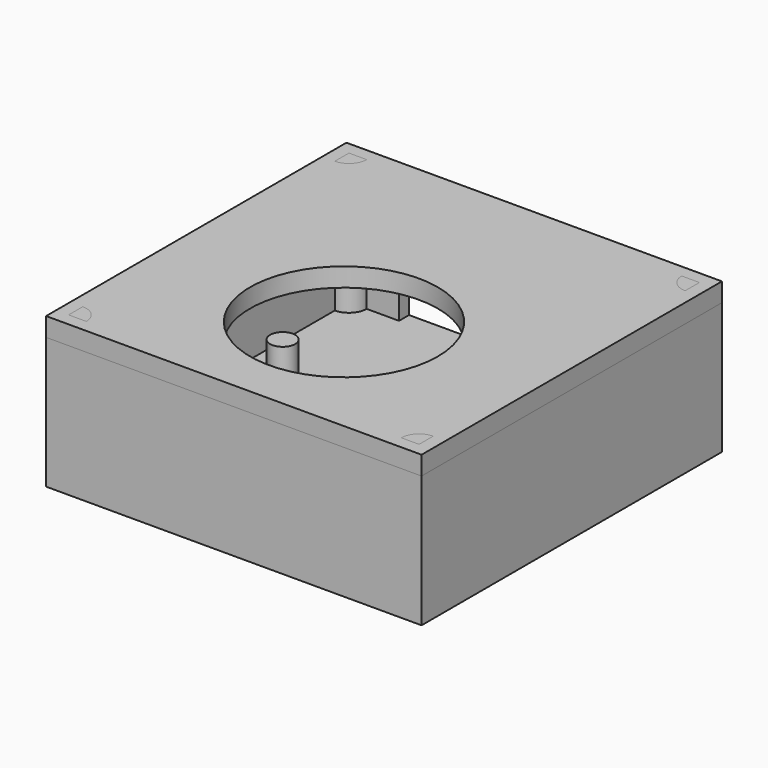
from build123d import *

# Parameters (mm, degrees)
F0_R     = 1
F0_W     = 20
F0_H     = 1
F1_DEPTH = 1.5
F2_DEPTH = 3
F3_DEPTH = 9
F4_W     = 20
F4_H     = 1
F4_R     = 7.5
F5_DEPTH = 1.5
F6_DEPTH = 10.5
F7_DEPTH = 25
F8_DEPTH = 5
F13_R    = 2


with BuildPart() as f1:
    # F0 (on Top) → F1 (new body)
    with BuildSketch(Plane.XY):
        with BuildLine():
            Line((25, -1), (5, -1))
            Line((5, -1), (2.4142135624, -1))
            ThreePointArc((2.4142135624, -1), (2, -2), (1, -2.4142135624))
            Line((1, -2.4142135624), (1, -27.5857864376))
            ThreePointArc((1, -27.5857864376), (2, -28), (2.4142135624, -29))
            Line((2.4142135624, -29), (27.5857864376, -29))
            ThreePointArc((27.5857864376, -29), (28, -28), (29, -27.5857864376))
            Line((29, -27.5857864376), (29, -2.4142135624))
            ThreePointArc((29, -2.4142135624), (28, -2), (27.5857864376, -1))
            Line((27.5857864376, -1), (25, -1))
        make_face()
        with Locations((4.5, -26)):
            Circle(F0_R, mode=Mode.SUBTRACT)
        with Locations((25.5, -26)):
            Circle(F0_R, mode=Mode.SUBTRACT)
        with Locations((4.5, -12)):
            Circle(F0_R, mode=Mode.SUBTRACT)
        with Locations((25.5, -12)):
            Circle(F0_R, mode=Mode.SUBTRACT)
        with BuildLine():
            Line((27.5857864376, -29), (2.4142135624, -29))
            ThreePointArc((2.4142135624, -29), (2.3065629649, -29.5411961001), (2, -30))
            Line((2, -30), (28, -30))
            ThreePointArc((28, -30), (27.6934370351, -29.5411961001), (27.5857864376, -29))
        make_face()
        with BuildLine():
            ThreePointArc((1, -2.4142135624), (0.4588038999, -2.3065629649), (0, -2))
            Line((0, -2), (0, -28))
            ThreePointArc((0, -28), (0.4588038999, -27.6934370351), (1, -27.5857864376))
            Line((1, -27.5857864376), (1, -2.4142135624))
        make_face()
        with BuildLine():
            Line((30, -28), (30, -2))
            ThreePointArc((30, -2), (29.5411961001, -2.3065629649), (29, -2.4142135624))
            Line((29, -2.4142135624), (29, -27.5857864376))
            ThreePointArc((29, -27.5857864376), (29.5411961001, -27.6934370351), (30, -28))
        make_face()
        with Locations((15, -0.5)):
            Rectangle(F0_W, F0_H)
        with BuildLine():
            ThreePointArc((1, -27.5857864376), (0.4588038999, -27.6934370351), (0, -28))
            Line((0, -28), (0, -30))
            Line((0, -30), (2, -30))
            ThreePointArc((2, -30), (2.3065629649, -29.5411961001), (2.4142135624, -29))
            Line((2.4142135624, -29), (1, -29))
            Line((1, -29), (1, -27.5857864376))
        make_face()
        with BuildLine():
            Line((30, -30), (30, -28))
            ThreePointArc((30, -28), (29.5411961001, -27.6934370351), (29, -27.5857864376))
            Line((29, -27.5857864376), (29, -29))
            Line((29, -29), (27.5857864376, -29))
            ThreePointArc((27.5857864376, -29), (27.6934370351, -29.5411961001), (28, -30))
            Line((28, -30), (30, -30))
        make_face()
        with BuildLine():
            ThreePointArc((2.4142135624, -1), (2.3065629649, -0.4588038999), (2, 0))
            Line((2, 0), (0, 0))
            Line((0, 0), (0, -2))
            ThreePointArc((0, -2), (0.4588038999, -2.3065629649), (1, -2.4142135624))
            Line((1, -2.4142135624), (1, -1))
            Line((1, -1), (2.4142135624, -1))
        make_face()
        with BuildLine():
            Line((30, 0), (28, 0))
            ThreePointArc((28, 0), (27.6934370351, -0.4588038999), (27.5857864376, -1))
            Line((27.5857864376, -1), (29, -1))
            Line((29, -1), (29, -2.4142135624))
            ThreePointArc((29, -2.4142135624), (29.5411961001, -2.3065629649), (30, -2))
            Line((30, -2), (30, 0))
        make_face()
        with Locations((4.5, -12)):
            Circle(F0_R)
        with Locations((4.5, -26)):
            Circle(F0_R)
        with Locations((25.5, -26)):
            Circle(F0_R)
        with Locations((25.5, -12)):
            Circle(F0_R)
        with BuildLine():
            Line((28, 0), (25, 0))
            Line((25, 0), (25, -1))
            Line((25, -1), (27.5857864376, -1))
            ThreePointArc((27.5857864376, -1), (27.6934370351, -0.4588038999), (28, 0))
        make_face()
        with BuildLine():
            Line((5, -1), (5, 0))
            Line((5, 0), (2, 0))
            ThreePointArc((2, 0), (2.3065629649, -0.4588038999), (2.4142135624, -1))
            Line((2.4142135624, -1), (5, -1))
        make_face()
        with BuildLine():
            ThreePointArc((1, -2.4142135624), (2, -2), (2.4142135624, -1))
            Line((2.4142135624, -1), (1, -1))
            Line((1, -1), (1, -2.4142135624))
        make_face()
        with BuildLine():
            ThreePointArc((2.4142135624, -29), (2, -28), (1, -27.5857864376))
            Line((1, -27.5857864376), (1, -29))
            Line((1, -29), (2.4142135624, -29))
        make_face()
        with BuildLine():
            Line((29, -29), (29, -27.5857864376))
            ThreePointArc((29, -27.5857864376), (28, -28), (27.5857864376, -29))
            Line((27.5857864376, -29), (29, -29))
        make_face()
        with BuildLine():
            Line((29, -1), (27.5857864376, -1))
            ThreePointArc((27.5857864376, -1), (28, -2), (29, -2.4142135624))
            Line((29, -2.4142135624), (29, -1))
        make_face()
    extrude(amount=-F1_DEPTH)

    # F0 (on Top) → F2 (join)
    with BuildSketch(Plane.XY):
        with Locations((4.5, -12)):
            Circle(F0_R)
        with Locations((25.5, -12)):
            Circle(F0_R)
        with Locations((25.5, -26)):
            Circle(F0_R)
        with Locations((4.5, -26)):
            Circle(F0_R)
    extrude(amount=F2_DEPTH)

    # F0 (on Top) → F3 (join)
    with BuildSketch(Plane.XY):
        with BuildLine():
            ThreePointArc((1, -27.5857864376), (0.4588038999, -27.6934370351), (0, -28))
            Line((0, -28), (0, -30))
            Line((0, -30), (2, -30))
            ThreePointArc((2, -30), (2.3065629649, -29.5411961001), (2.4142135624, -29))
            Line((2.4142135624, -29), (1, -29))
            Line((1, -29), (1, -27.5857864376))
        make_face()
        with BuildLine():
            Line((27.5857864376, -29), (2.4142135624, -29))
            ThreePointArc((2.4142135624, -29), (2.3065629649, -29.5411961001), (2, -30))
            Line((2, -30), (28, -30))
            ThreePointArc((28, -30), (27.6934370351, -29.5411961001), (27.5857864376, -29))
        make_face()
        with BuildLine():
            Line((30, -30), (30, -28))
            ThreePointArc((30, -28), (29.5411961001, -27.6934370351), (29, -27.5857864376))
            Line((29, -27.5857864376), (29, -29))
            Line((29, -29), (27.5857864376, -29))
            ThreePointArc((27.5857864376, -29), (27.6934370351, -29.5411961001), (28, -30))
            Line((28, -30), (30, -30))
        make_face()
        with BuildLine():
            Line((30, -28), (30, -2))
            ThreePointArc((30, -2), (29.5411961001, -2.3065629649), (29, -2.4142135624))
            Line((29, -2.4142135624), (29, -27.5857864376))
            ThreePointArc((29, -27.5857864376), (29.5411961001, -27.6934370351), (30, -28))
        make_face()
        with BuildLine():
            Line((30, 0), (28, 0))
            ThreePointArc((28, 0), (27.6934370351, -0.4588038999), (27.5857864376, -1))
            Line((27.5857864376, -1), (29, -1))
            Line((29, -1), (29, -2.4142135624))
            ThreePointArc((29, -2.4142135624), (29.5411961001, -2.3065629649), (30, -2))
            Line((30, -2), (30, 0))
        make_face()
        with BuildLine():
            Line((28, 0), (25, 0))
            Line((25, 0), (25, -1))
            Line((25, -1), (27.5857864376, -1))
            ThreePointArc((27.5857864376, -1), (27.6934370351, -0.4588038999), (28, 0))
        make_face()
        with BuildLine():
            Line((5, -1), (5, 0))
            Line((5, 0), (2, 0))
            ThreePointArc((2, 0), (2.3065629649, -0.4588038999), (2.4142135624, -1))
            Line((2.4142135624, -1), (5, -1))
        make_face()
        with BuildLine():
            ThreePointArc((2.4142135624, -1), (2.3065629649, -0.4588038999), (2, 0))
            Line((2, 0), (0, 0))
            Line((0, 0), (0, -2))
            ThreePointArc((0, -2), (0.4588038999, -2.3065629649), (1, -2.4142135624))
            Line((1, -2.4142135624), (1, -1))
            Line((1, -1), (2.4142135624, -1))
        make_face()
        with BuildLine():
            ThreePointArc((1, -2.4142135624), (0.4588038999, -2.3065629649), (0, -2))
            Line((0, -2), (0, -28))
            ThreePointArc((0, -28), (0.4588038999, -27.6934370351), (1, -27.5857864376))
            Line((1, -27.5857864376), (1, -2.4142135624))
        make_face()
    extrude(amount=F3_DEPTH)

    # F0 (on Top) → F6 (join)
    with BuildSketch(Plane.XY):
        with BuildLine():
            ThreePointArc((1, -2.4142135624), (2, -2), (2.4142135624, -1))
            Line((2.4142135624, -1), (1, -1))
            Line((1, -1), (1, -2.4142135624))
        make_face()
        with BuildLine():
            ThreePointArc((2.4142135624, -29), (2, -28), (1, -27.5857864376))
            Line((1, -27.5857864376), (1, -29))
            Line((1, -29), (2.4142135624, -29))
        make_face()
        with BuildLine():
            Line((29, -29), (29, -27.5857864376))
            ThreePointArc((29, -27.5857864376), (28, -28), (27.5857864376, -29))
            Line((27.5857864376, -29), (29, -29))
        make_face()
        with BuildLine():
            Line((29, -1), (27.5857864376, -1))
            ThreePointArc((27.5857864376, -1), (28, -2), (29, -2.4142135624))
            Line((29, -2.4142135624), (29, -1))
        make_face()
    extrude(amount=F6_DEPTH)

    # F7 (cut): faces of the model
    f7_faces = [f1.faces().sort_by_distance(p)[0] for p in [
        (28.3997891226, -1.6002108774, 10.5),
        (1.6002108774, -1.6002108774, 10.5),
        (1.6002108774, -28.3997891226, 10.5),
        (28.3997891226, -28.3997891226, 10.5),
    ]]
    extrude(f7_faces, amount=F7_DEPTH, mode=Mode.SUBTRACT)


with BuildPart() as f5:
    # F4 (on face) → F5 (new body)
    with BuildSketch(Plane.XY.offset(9)):
        with Locations((15, -0.5)):
            Rectangle(F4_W, F4_H)
        Polygon((30, 0), (25, 0), (25, -1), (27.5857864376, -1), (29, -1), (29, -2.4142135624), (29, -27.5857864376), (29, -29), (27.5857864376, -29), (2.4142135624, -29), (1, -29), (1, -27.5857864376), (1, -2.4142135624), (1, -1), (2.4142135624, -1), (5, -1), (5, 0), (0, 0), (0, -30), (30, -30), align=None)
        with BuildLine():
            Line((27.5857864376, -1), (25, -1))
            Line((25, -1), (5, -1))
            Line((5, -1), (2.4142135624, -1))
            ThreePointArc((2.4142135624, -1), (2, -2), (1, -2.4142135624))
            Line((1, -2.4142135624), (1, -27.5857864376))
            ThreePointArc((1, -27.5857864376), (2, -28), (2.4142135624, -29))
            Line((2.4142135624, -29), (27.5857864376, -29))
            ThreePointArc((27.5857864376, -29), (28, -28), (29, -27.5857864376))
            Line((29, -27.5857864376), (29, -2.4142135624))
            ThreePointArc((29, -2.4142135624), (28, -2), (27.5857864376, -1))
        make_face()
        with Locations((15, -19)):
            Circle(F4_R, mode=Mode.SUBTRACT)
    extrude(amount=F5_DEPTH)


with BuildPart() as f8:
    # F4 (on face) → F8 (new body)
    with BuildSketch(Plane.XY.offset(9)):
        with Locations((15, -0.5)):
            Rectangle(F4_W, F4_H)
    extrude(amount=-F8_DEPTH)


with BuildPart() as f11:
    # F9 (on Right) → F11 (revolve)
    with BuildSketch(Plane.YZ):
        with BuildLine():
            Line((15.2258750796, -40.7793708146), (25.2258750796, -40.7793708146))
            ThreePointArc((25.2258750796, -40.7793708146), (21.3738474037, -35.9129389037), (15.7530112624, -38.5447591543))
            Line((15.7530112624, -38.5447591543), (9.7055286169, -38.5447591543))
            Line((9.7055286169, -38.5447591543), (9.7055286169, -36.1464507878))
            Line((9.7055286169, -36.1464507878), (5.4970784113, -36.1464507878))
            Line((5.4970784113, -36.1464507878), (5.4970784113, -40.7793708146))
            Line((5.4970784113, -40.7793708146), (15.2258750796, -40.7793708146))
        make_face()
    revolve(axis=Axis((0, 20.2258750796, -40.7793708146), (0, 1, 0)))


with BuildPart() as f12:
    # F10 (on Right) → F12 (revolve)
    with BuildSketch(Plane.YZ):
        with BuildLine():
            ThreePointArc((18.9868118614, -35.8321774343), (23.3636113326, -36.7588470668), (25.3258750796, -40.7793708146))
            Line((25.3258750796, -40.7793708146), (26.2448396534, -40.7793708146))
            Line((26.2448396534, -40.7793708146), (30.2728638053, -40.7793708146))
            Line((30.2728638053, -40.7793708146), (30.2728638053, -38.8744622469))
            Line((30.2728638053, -38.8744622469), (26.2448396534, -38.8744622469))
            Line((26.2448396534, -38.8744622469), (26.2448396534, -34.7860343754))
            Line((26.2448396534, -34.7860343754), (18.9868118614, -34.7860343754))
            Line((18.9868118614, -34.7860343754), (18.9868118614, -35.8321774343))
        make_face()
    revolve(axis=Axis((0, 28.2588517293, -40.7793708146), (0, 1, 0)))

    # F13
    f13_edges = [f12.edges().sort_by_distance(p)[0] for p in [
        (0, 26.24484, -42.684279),
    ]]
    fillet(f13_edges, radius=F13_R)


solid = Compound([f1.part, f5.part, f8.part])
